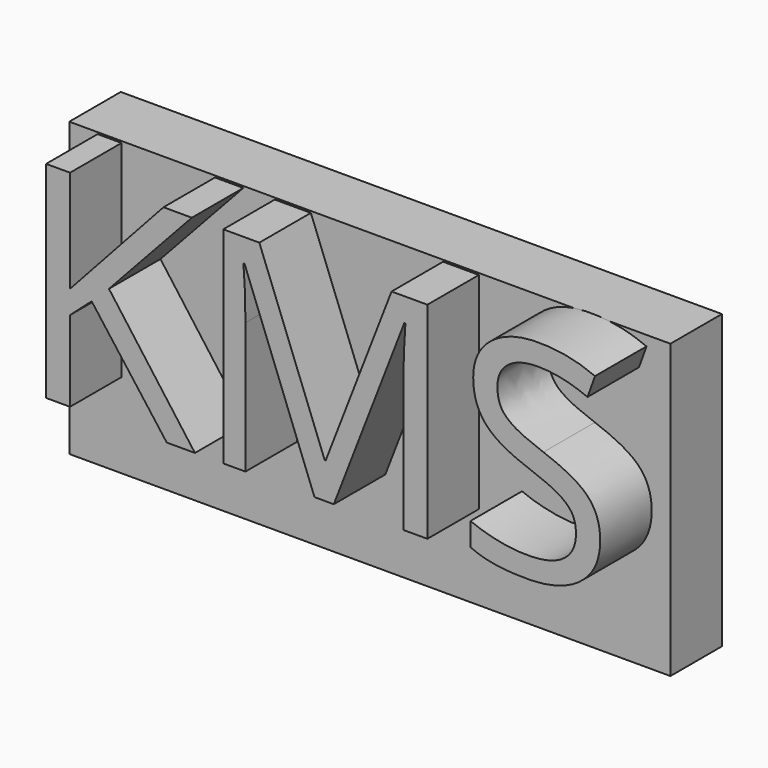
from build123d import *

# Parameters (mm, degrees)
F0_W         = 93.3757275343
F0_H         = 45.4434677958
F1_DEPTH     = 10
F2_TEXT_SIZE = 44.8416489997
F3_DEPTH     = 10


# Not quite as in the source:
# - Text() gives the source's letters only with a copy of the font that has no kerning and outlines rounded to 1/6400 em; it was checked with that copy


with BuildPart() as f1:
    # F0 (on Front) → F1 (new body)
    with BuildSketch(Plane.XZ):
        with Locations((46.6878637671, 22.7217338979)):
            Rectangle(F0_W, F0_H)
    extrude(amount=F1_DEPTH)

    # F2 (on face) → F3 (join)
    with BuildSketch(Plane.XZ.offset(10)):
        with Locations((0, 13.157480516)):
            Text('KMS', F2_TEXT_SIZE, font='Open Sans', text_align=(TextAlign.LEFT, TextAlign.BOTTOM))
    extrude(amount=F3_DEPTH)


solid = f1.part
